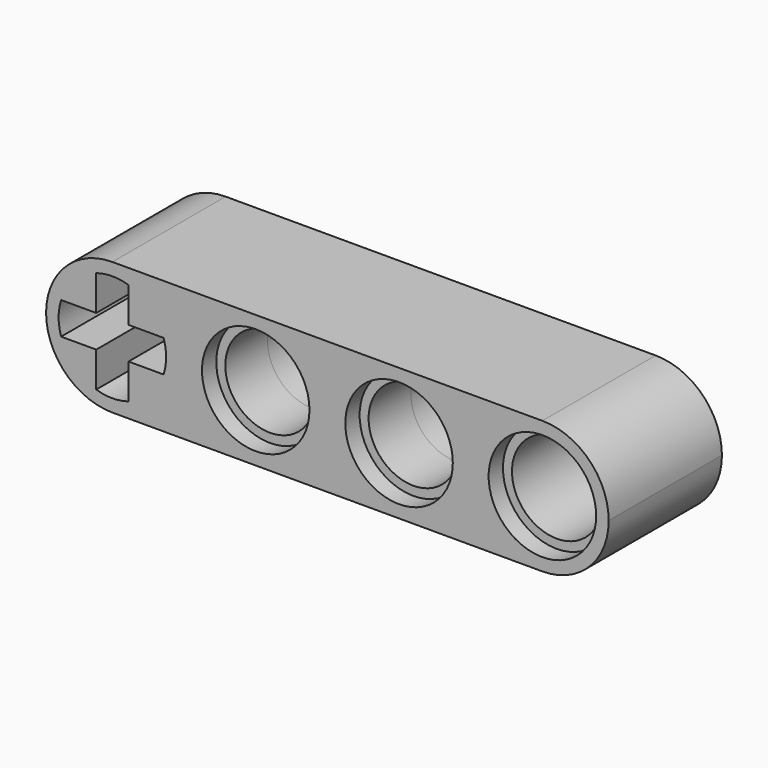
from build123d import *

# Parameters (mm, degrees)
F0_W     = 31.4
F0_H     = 7.4
F0_R     = 3
F1_DEPTH = 3.95
F0_R_2   = 2.499
F2_DEPTH = 2.95
F3_R     = 3.69999


# Not quite as in the source:
# - a fillet or chamfer is up to 0.001 mm smaller than in the source, because OpenCascade refuses the exact size


with BuildPart() as f1:
    # F0 (on Front) → F1 (new body, symmetric)
    with BuildSketch(Plane.XZ):
        Rectangle(F0_W, F0_H)
        with BuildLine():
            ThreePointArc((-12.9, 2.8618176043), (-12, 3), (-11.1, 2.8618176043))
            Line((-11.1, 2.8618176043), (-11.1, 0.9))
            Line((-11.1, 0.9), (-9.1381823957, 0.9))
            ThreePointArc((-9.1381823957, 0.9), (-9, 0), (-9.1381823957, -0.9))
            Line((-9.1381823957, -0.9), (-11.1, -0.9))
            Line((-11.1, -0.9), (-11.1, -2.8618176043))
            ThreePointArc((-11.1, -2.8618176043), (-12, -3), (-12.9, -2.8618176043))
            Line((-12.9, -2.8618176043), (-12.9, -0.9))
            Line((-12.9, -0.9), (-14.8618176043, -0.9))
            ThreePointArc((-14.8618176043, -0.9), (-15, 0), (-14.8618176043, 0.9))
            Line((-14.8618176043, 0.9), (-12.9, 0.9))
            Line((-12.9, 0.9), (-12.9, 2.8618176043))
        make_face(mode=Mode.SUBTRACT)
        with Locations((-4, 0)):
            Circle(F0_R, mode=Mode.SUBTRACT)
        with Locations((4, 0)):
            Circle(F0_R, mode=Mode.SUBTRACT)
        with Locations((12, 0)):
            Circle(F0_R, mode=Mode.SUBTRACT)
    extrude(amount=F1_DEPTH, both=True)

    # F0 (on Front) → F2 (join, symmetric)
    with BuildSketch(Plane.XZ):
        with Locations((-4, 0)):
            Circle(F0_R)
        with Locations((-4, 0)):
            Circle(F0_R_2, mode=Mode.SUBTRACT)
        with Locations((4, 0)):
            Circle(F0_R)
        with Locations((4, 0)):
            Circle(F0_R_2, mode=Mode.SUBTRACT)
        with Locations((12, 0)):
            Circle(F0_R)
        with Locations((12, 0)):
            Circle(F0_R_2, mode=Mode.SUBTRACT)
    extrude(amount=F2_DEPTH, both=True)

    # F3 (radius 3.7 in the source; OpenCascade refuses exactly that, so slightly less here)
    f3_edges = [f1.edges().sort_by_distance(p)[0] for p in [
        (-15.7, 0, 3.7),
        (-15.7, 0, -3.7),
        (15.7, 0, 3.7),
        (15.7, 0, -3.7),
    ]]
    fillet(f3_edges, radius=F3_R)


solid = f1.part
